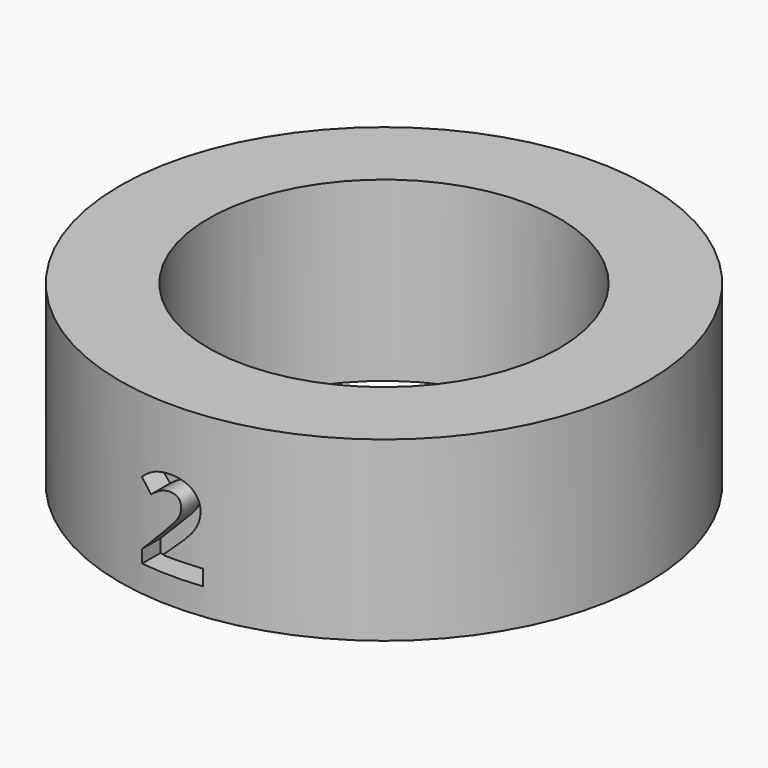
from build123d import *

# Parameters (mm, degrees)
F0_R         = 14.9
F0_R_2       = 9.9
F1_DEPTH     = 10
F3_TEXT_SIZE = 6.9444444444
F4_DEPTH     = 1.5


# Not quite as in the source:
# - Text() gives the source's letters only with a copy of the font that has no kerning and outlines rounded to 1/6400 em; it was checked with that copy


with BuildPart() as f1:
    # F0 (on Top) → F1 (new body)
    with BuildSketch(Plane.XY):
        Circle(F0_R)
        Circle(F0_R_2, mode=Mode.SUBTRACT)
    extrude(amount=F1_DEPTH)

    # F3 (on offset) → F4 (cut)
    with BuildSketch(Plane.XZ.offset(15)):
        with Locations((-2.0968967014, 1.500000013)):
            Text('2', F3_TEXT_SIZE, font='Open Sans', font_style=FontStyle.BOLD, text_align=(TextAlign.LEFT, TextAlign.BOTTOM))
    extrude(amount=-F4_DEPTH, mode=Mode.SUBTRACT)


solid = f1.part
